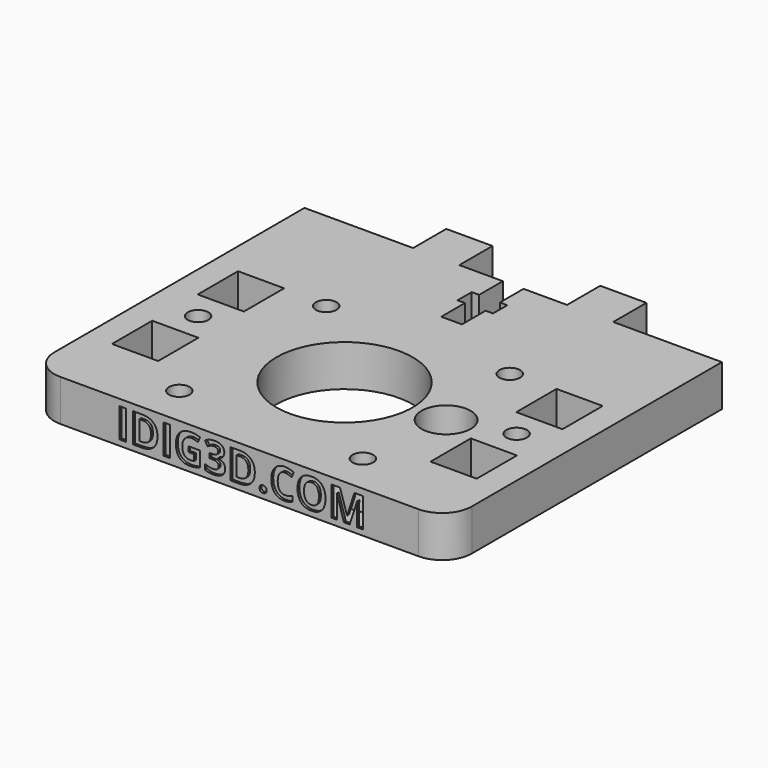
from build123d import *

# Parameters (mm, degrees)
F0_W         = 7.8
F0_H         = 7
F0_H_2       = 8.5
F0_R         = 1.75
F0_R_2       = 4.15
F0_R_3       = 11.5
F1_DEPTH     = 7
F2_ANGLE     = 180
F3_TEXT_SIZE = 6.9444444444
F4_DEPTH     = 0.4


# Not quite as in the source:
# - Text() gives the source's letters only with a copy of the font that has no kerning and outlines rounded to 1/6400 em; it was checked with that copy


with BuildPart() as f1:
    # F0 (on Top) → F1 (new body)
    with BuildSketch(Plane.XY):
        with Locations((-13, 32.4)):
            Rectangle(F0_W, F0_H)
        with Locations((13, 32.4)):
            Rectangle(F0_W, F0_H)
        with BuildLine():
            Line((-16.9, 28.9), (-35.25, 28.9))
            Line((-35.25, 28.9), (-35.25, -23.9))
            ThreePointArc((-35.25, -23.9), (-33.7855339059, -27.4355339059), (-30.25, -28.9))
            Line((-30.25, -28.9), (30.25, -28.9))
            ThreePointArc((30.25, -28.9), (33.7855339059, -27.4355339059), (35.25, -23.9))
            Line((35.25, -23.9), (35.25, 28.9))
            Line((35.25, 28.9), (16.9, 28.9))
            Line((16.9, 28.9), (9.1, 28.9))
            Line((9.1, 28.9), (1.75, 28.9))
            Line((1.75, 28.9), (1.75, 23.9))
            Line((1.75, 23.9), (3, 23.9))
            Line((3, 23.9), (3, 20.9))
            Line((3, 20.9), (1.75, 20.9))
            Line((1.75, 20.9), (1.75, 15.9))
            Line((1.75, 15.9), (-1.75, 15.9))
            Line((-1.75, 15.9), (-1.75, 20.9))
            Line((-1.75, 20.9), (-3, 20.9))
            Line((-3, 20.9), (-3, 23.9))
            Line((-3, 23.9), (-1.75, 23.9))
            Line((-1.75, 23.9), (-1.75, 28.9))
            Line((-1.75, 28.9), (-9.1, 28.9))
            Line((-9.1, 28.9), (-16.9, 28.9))
        make_face()
        with Locations((-26.9, -13.05)):
            Rectangle(F0_W, F0_H_2, mode=Mode.SUBTRACT)
        with Locations((-15.5, -22.2)):
            Circle(F0_R, mode=Mode.SUBTRACT)
        with Locations((-26.9, -4)):
            Circle(F0_R, mode=Mode.SUBTRACT)
        with Locations((-17.15, -6.7)):
            Circle(F0_R_2, mode=Mode.SUBTRACT)
        with Locations((15.5, -22.2)):
            Circle(F0_R, mode=Mode.SUBTRACT)
        with Locations((26.9, -13.05)):
            Rectangle(F0_W, F0_H_2, mode=Mode.SUBTRACT)
        with Locations((0, -6.7)):
            Circle(F0_R_3, mode=Mode.SUBTRACT)
        with Locations((26.9, -4)):
            Circle(F0_R, mode=Mode.SUBTRACT)
        with Locations((-26.9, 5.05)):
            Rectangle(F0_W, F0_H_2, mode=Mode.SUBTRACT)
        with Locations((-15.5, 8.8)):
            Circle(F0_R, mode=Mode.SUBTRACT)
        with Locations((15.5, 8.8)):
            Circle(F0_R, mode=Mode.SUBTRACT)
        with Locations((26.9, 5.05)):
            Rectangle(F0_W, F0_H_2, mode=Mode.SUBTRACT)
    extrude(amount=F1_DEPTH)


with BuildPart() as f1_1:
    # F2: moved
    add(f1.part.rotate(Axis((0, -10.6412042961, 0), (0, 1, 0)), F2_ANGLE))

    # F3 (on face) → F4 (cut)
    with BuildSketch(Plane.XZ.offset(28.9)):
        with Locations((-20.8642578125, -6.0504147588)):
            Text('IDIG3D.COM', F3_TEXT_SIZE, font='Open Sans', font_style=FontStyle.BOLD, text_align=(TextAlign.LEFT, TextAlign.BOTTOM))
    extrude(amount=-F4_DEPTH, mode=Mode.SUBTRACT)


solid = f1_1.part
